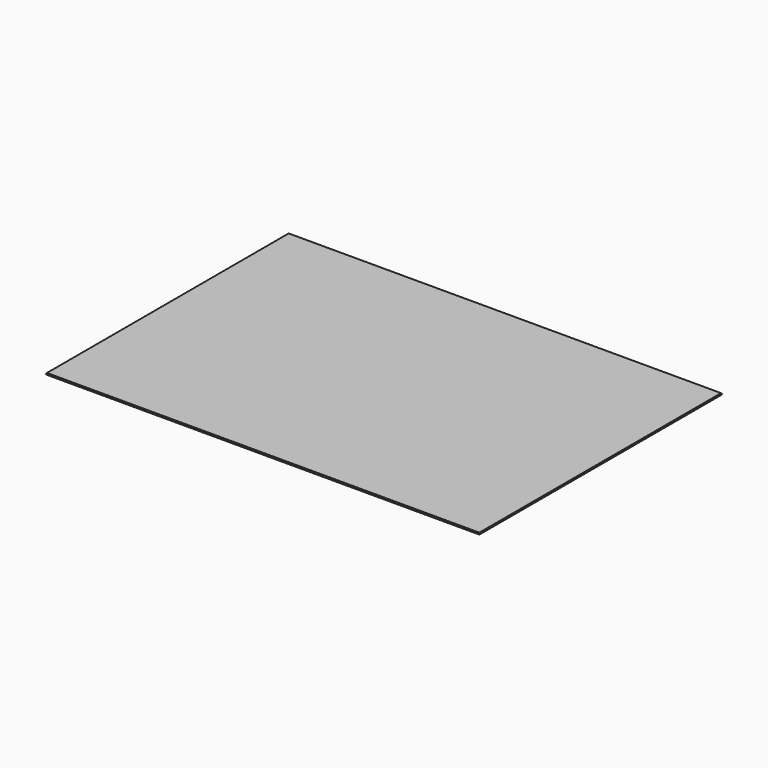
from build123d import *

# Parameters (mm, degrees)
F0_W     = 500
F0_H     = 350
F1_DEPTH = 2
F2_SIZE  = 0.99999


# Not quite as in the source:
# - a fillet or chamfer is up to 0.001 mm smaller than in the source, because OpenCascade refuses the exact size


with BuildPart() as f1:
    # F0 (on Top) → F1 (new body)
    with BuildSketch(Plane.XY):
        Rectangle(F0_W, F0_H)
    extrude(amount=F1_DEPTH)

    # F2 (size 1 in the source; OpenCascade refuses exactly that, so slightly less here)
    f2_edges = [f1.edges().sort_by_distance(p)[0] for p in [
        (0, 175, 0),
        (-250, 0, 0),
        (-250, 0, 2),
        (0, 175, 2),
        (250, 0, 0),
        (0, -175, 2),
        (250, 0, 2),
        (0, -175, 0),
        (-250, -175, 1),
        (-250, 175, 1),
        (250, 175, 1),
        (250, -175, 1),
    ]]
    chamfer(f2_edges, length=F2_SIZE)


solid = f1.part
